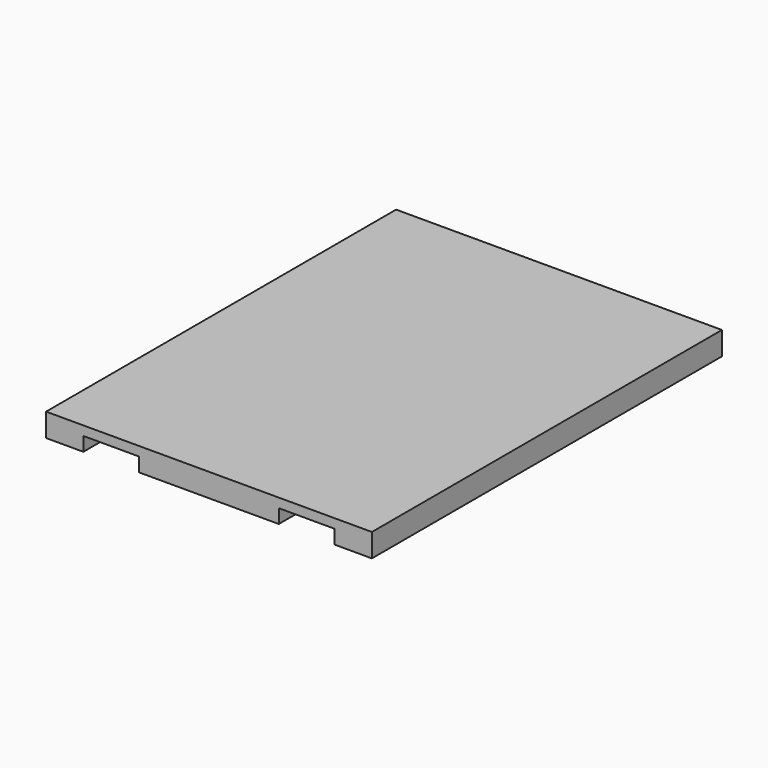
from build123d import *

# Parameters (mm, degrees)
F0_W        = 35
F0_H        = 47
F1_DEPTH    = 2.5
F2_W        = 6
F2_H        = 1.5
F3_DEPTH    = 4
F4_W        = 15
F4_H        = 4
F5_DEPTH    = 2
F6_T1_DEPTH = 35
F7_W        = 11
F7_H        = 1
F8_DEPTH    = 1


# Not quite as in the source:
# - a fillet or chamfer that OpenCascade refuses, or shapes differently, is made with other operations: its cross-section is extruded or revolved along the edge and cut away or added


with BuildPart() as f1:
    # F0 (on Top) → F1 (new body)
    with BuildSketch(Plane.XY):
        with Locations((6.565169383, -0.3048535436)):
            Rectangle(F0_W, F0_H)
    extrude(amount=F1_DEPTH)

    # F2 (on face) → F3 (cut)
    with BuildSketch(Plane.XZ.offset(23.8048535436)):
        with Locations((-3.934830617, 0.75)):
            Rectangle(F2_W, F2_H)
        with Locations((17.065169383, 0.75)):
            Rectangle(F2_W, F2_H)
    extrude(amount=-F3_DEPTH, mode=Mode.SUBTRACT)

    # F4 (on face) → F5 (join)
    with BuildSketch(Plane(origin=(0, 0, 0), x_dir=(1, 0, 0), z_dir=(0, 0, -1))):
        with Locations((6.565169383, -21.1951464564)):
            Rectangle(F4_W, F4_H)
    extrude(amount=F5_DEPTH)

    # F6: fillet of radius 5 on 1 edges, made by hand

    # F6_s2 → F6_t1 (cut)
    with BuildSketch(Plane.YZ.offset(-10.934830617)):
        with BuildLine():
            ThreePointArc((19.1951464564, 0), (20.9590784789, -1.472135955), (23.1951464564, -2))
            Line((23.1951464564, -2), (19.1951464564, -2))
            Line((19.1951464564, -2), (19.1951464564, 0))
        make_face()
    extrude(amount=F6_T1_DEPTH, mode=Mode.SUBTRACT)

    # F7 (on face) → F8 (cut)
    with BuildSketch(Plane(origin=(0, 23.1951464564, 0), x_dir=(-1, 0, 0), z_dir=(0, 1, 0))):
        with Locations((-6.565169383, -1)):
            Rectangle(F7_W, F7_H)
    extrude(amount=-F8_DEPTH, mode=Mode.SUBTRACT)


solid = f1.part
